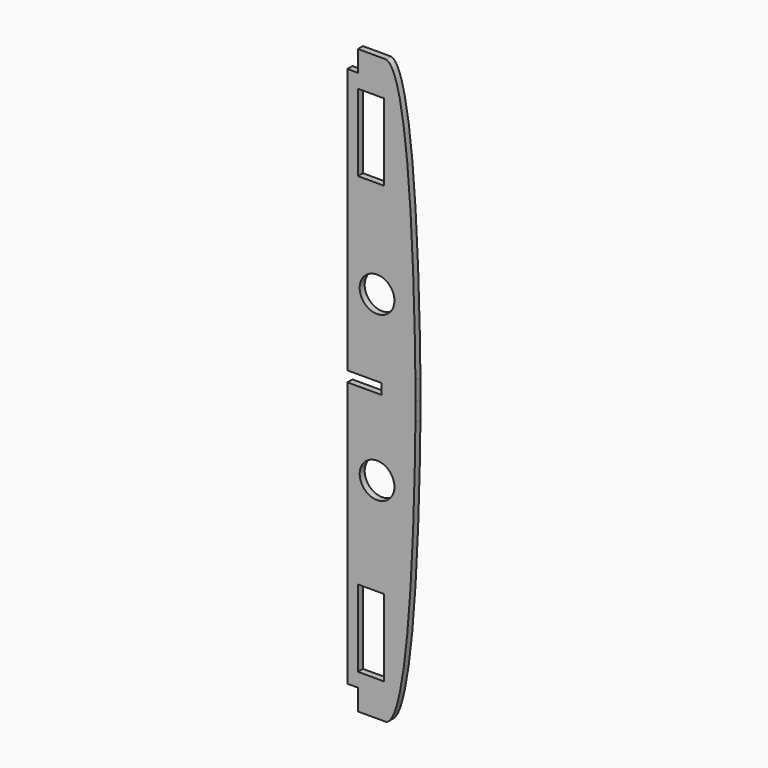
from build123d import *

# Parameters (mm, degrees)
F0_R     = 16.5575031532
F0_W     = 25.0224173069
F0_H     = 73.3505785465
F1_DEPTH = 6


# Not quite as in the source:
# - a feature names something its author has since deleted; it is built from what else it names


with BuildPart() as f1:
    # F0 (on Front) → F1 (new body)
    with BuildSketch(Plane.XZ):
        with BuildLine():
            add(Edge.make_bspline(
                [(248.9335625079, 167.3540463153), (272.5197521804, 160.3214966928), (276.1214780845, -32.6489303119), (276.7706038072, -92.8803390196)],
                knots=[0, 0, 0, 0, 236.7397799676, 236.7397799676, 236.7397799676, 236.7397799676], degree=3))
            Line((248.9335625079, 167.3540463153), (221.9335625079, 167.3540463153))
            Line((221.9335625079, 167.3540463153), (221.9335625079, 147.3540463153))
            Line((221.9335625079, 147.3540463153), (211.9335625079, 147.3540463153))
            Line((211.9335625079, 147.3540463153), (211.9335625079, -105.6459536847))
            Line((211.9335625079, -105.6459536847), (244.4335625079, -105.6459536847))
            Line((244.4335625079, -105.6459536847), (244.4335625079, -110.6459536847))
            Line((244.4335625079, -110.6459536847), (276.9335625079, -110.6459536847))
            add(Edge.make_bspline(
                [(276.7706038072, -92.8803390196), (276.8875933326, -103.7356227789), (276.9086779216, -110.279341705), (276.9335625079, -110.6459536847)],
                knots=[236.7397799676, 236.7397799676, 236.7397799676, 236.7397799676, 279.4065138826, 279.4065138826, 279.4065138826, 279.4065138826], degree=3))
        make_face()
        with Locations((240.1929050684, -32.5540304184)):
            Circle(F0_R, mode=Mode.SUBTRACT)
        with Locations((234.4716570738, 97.3541972034)):
            Rectangle(F0_W, F0_H, mode=Mode.SUBTRACT)
        with BuildLine():
            add(Edge.make_bspline(
                [(276.7706038072, -128.4115683497), (276.8875933326, -117.5562845905), (276.9086779216, -111.0125656644), (276.9335625079, -110.6459536847)],
                knots=[236.7397799677, 236.7397799677, 236.7397799677, 236.7397799677, 279.4065138826, 279.4065138826, 279.4065138826, 279.4065138826], degree=3))
            Line((276.9335625079, -110.6459536847), (244.4335625079, -110.6459536847))
            Line((244.4335625079, -110.6459536847), (244.4335625079, -115.6459536847))
            Line((244.4335625079, -115.6459536847), (211.9335625079, -115.6459536847))
            Line((211.9335625079, -115.6459536847), (211.9335625079, -368.6459536847))
            Line((211.9335625079, -368.6459536847), (221.9335625079, -368.6459536847))
            Line((221.9335625079, -368.6459536847), (221.9335625079, -388.6459536847))
            Line((221.9335625079, -388.6459536847), (248.9335625079, -388.6459536847))
            add(Edge.make_bspline(
                [(248.9335625079, -388.6459536847), (272.5197521804, -381.6134040622), (276.1214780845, -188.6429770574), (276.7706038072, -128.4115683497)],
                knots=[0, 0, 0, 0, 236.7397799677, 236.7397799677, 236.7397799677, 236.7397799677], degree=3))
        make_face()
        with Locations((234.4716570738, -318.6461045727)):
            Rectangle(F0_W, F0_H, mode=Mode.SUBTRACT)
        with Locations((240.1929050684, -188.737876951)):
            Circle(F0_R, mode=Mode.SUBTRACT)
    extrude(amount=F1_DEPTH)


solid = f1.part
